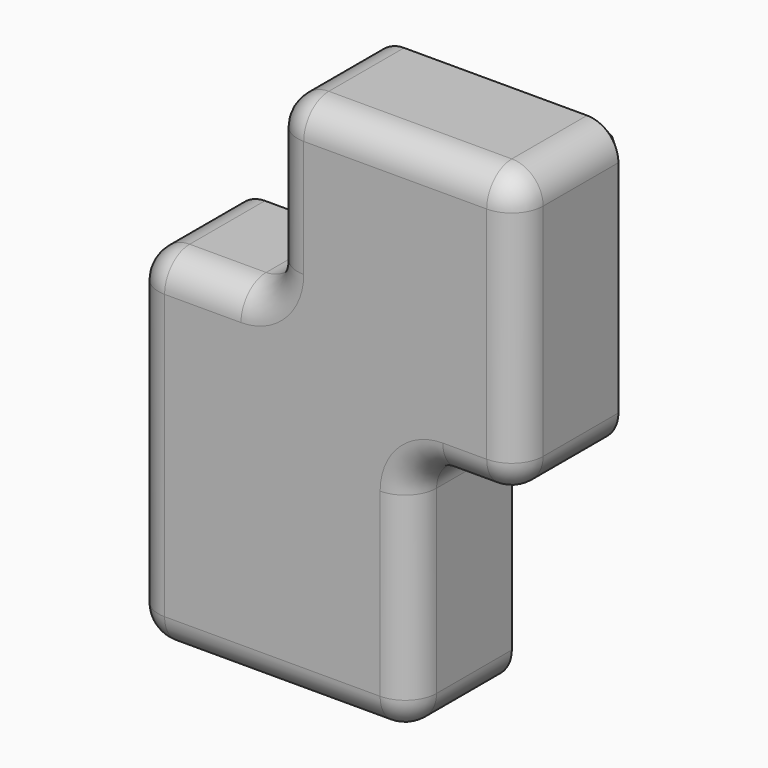
from build123d import *

# Parameters (mm, degrees)
F1_DEPTH = 25
F2_R     = 5
F3_SIZE  = 4.99999


# Not quite as in the source:
# - a fillet or chamfer is up to 0.001 mm smaller than in the source, because OpenCascade refuses the exact size


with BuildPart() as f1:
    # F0 (on Front) → F1 (new body)
    with BuildSketch(Plane.XZ):
        with BuildLine():
            Line((-4.1428460926, 16.4471715689), (-16.3246531785, 16.4471715689))
            ThreePointArc((-16.3246531785, 16.4471715689), (-19.8601870844, 14.9827054748), (-21.3246531785, 11.4471715689))
            Line((-21.3246531785, 11.4471715689), (-21.3246531785, -33.7977808714))
            ThreePointArc((-21.3246531785, -33.7977808714), (-19.8601870844, -37.3333147773), (-16.3246531785, -38.7977808714))
            Line((-16.3246531785, -38.7977808714), (18.0389609933, -38.7977808714))
            ThreePointArc((18.0389609933, -38.7977808714), (21.5744948992, -37.3333147773), (23.0389609933, -33.7977808714))
            Line((23.0389609933, -33.7977808714), (23.0389609933, -5))
            ThreePointArc((23.0389609933, -5), (24.5034270874, -1.4644660941), (28.0389609933, 0))
            Line((28.0389609933, 0), (35.034160018, 0))
            ThreePointArc((35.034160018, 0), (38.5696939239, 1.4644660941), (40.034160018, 5))
            Line((40.034160018, 5), (40.034160018, 40.125707984))
            ThreePointArc((40.034160018, 40.125707984), (38.5696939239, 43.6612418899), (35.034160018, 45.125707984))
            Line((35.034160018, 45.125707984), (5.8571539074, 45.125707984))
            ThreePointArc((5.8571539074, 45.125707984), (2.3216200015, 43.6612418899), (0.8571539074, 40.125707984))
            Line((0.8571539074, 40.125707984), (0.8571539074, 21.4471715689))
            ThreePointArc((0.8571539074, 21.4471715689), (-0.6073121866, 17.9116376629), (-4.1428460926, 16.4471715689))
        make_face()
    extrude(amount=F1_DEPTH)

    # F2
    f2_edges = [f1.edges().sort_by_distance(p)[0] for p in [
        (0.857154, -25, -38.797781),
    ]]
    fillet(f2_edges, radius=F2_R)

    # F3 (size 5 in the source; OpenCascade refuses exactly that, so slightly less here)
    f3_edges = [f1.edges().sort_by_distance(p)[0] for p in [
        (20.445657, 0, 45.125708),
        (2.32162, 0, 43.661242),
        (0.857154, 0, 30.78644),
        (-0.607312, 0, 17.911638),
        (-10.23375, 0, 16.447172),
        (-19.860187, 0, 14.982705),
        (-21.324653, 0, -11.175305),
        (-19.860187, 0, -37.333315),
        (0.857154, 0, -38.797781),
        (21.574495, 0, -37.333315),
        (23.038961, 0, -19.39889),
        (24.503427, 0, -1.464466),
        (31.536561, 0, 0),
        (38.569694, 0, 1.464466),
        (40.03416, 0, 22.562854),
        (38.569694, 0, 43.661242),
    ]]
    chamfer(f3_edges, length=F3_SIZE)


solid = f1.part
